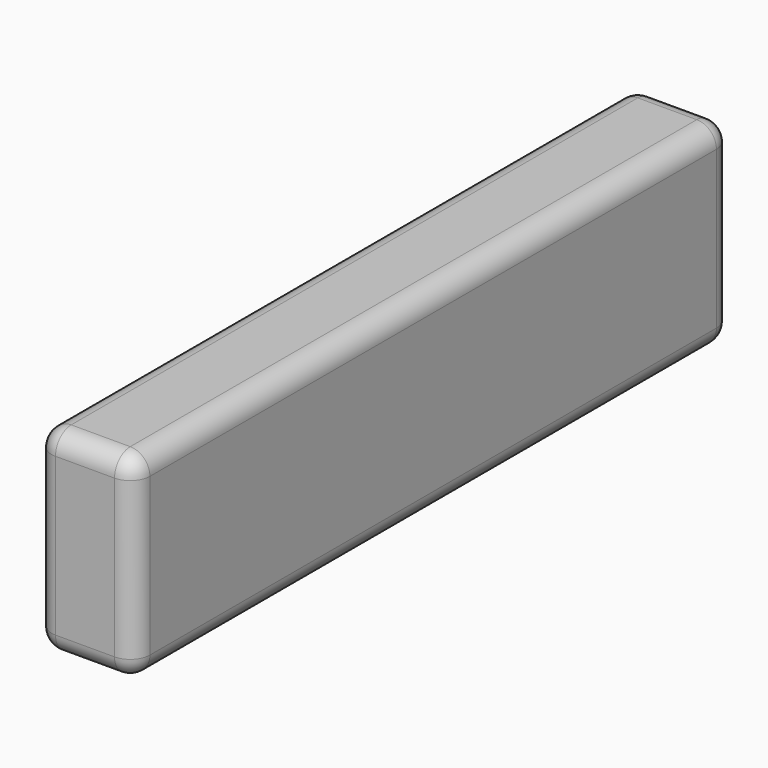
from build123d import *

# Parameters (mm, degrees)
F0_W     = 25
F0_H     = 50
F1_DEPTH = 190
F2_R     = 5


with BuildPart() as f1:
    # F0 (on Front) → F1 (new body)
    with BuildSketch(Plane.XZ):
        with Locations((12.5, 25)):
            Rectangle(F0_W, F0_H)
    extrude(amount=F1_DEPTH)

    # F2
    f2_edges = [f1.edges().sort_by_distance(p)[0] for p in [
        (25, -190, 25),
        (12.5, -190, 50),
        (0, -190, 25),
        (12.5, -190, 0),
        (0, -95, 50),
        (12.5, 0, 50),
        (25, -95, 0),
        (0, -95, 0),
        (12.5, 0, 0),
        (25, -95, 50),
        (0, 0, 25),
        (25, 0, 25),
    ]]
    fillet(f2_edges, radius=F2_R)


solid = f1.part
